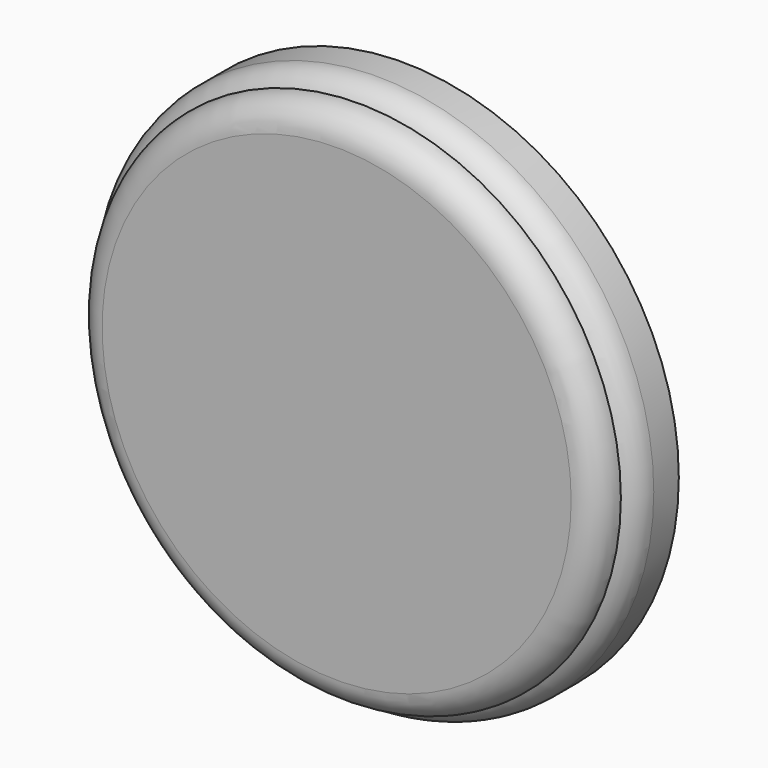
from build123d import *

# Parameters (mm, degrees)
F0_R     = 50
F1_DEPTH = 10
F2_R     = 47.5
F3_DEPTH = 5


# Not quite as in the source:
# - a fillet or chamfer that OpenCascade refuses, or shapes differently, is made with other operations: its cross-section is extruded or revolved along the edge and cut away or added


with BuildPart() as f1:
    # F0 (on Front) → F1 (new body)
    with BuildSketch(Plane.XZ):
        Circle(F0_R)
    extrude(amount=F1_DEPTH)

    # F2 (on face) → F3 (join)
    with BuildSketch(Plane.XZ.offset(10)):
        Circle(F2_R)
    extrude(amount=F3_DEPTH)

    # F4: fillet of radius 5 on 2 edges, made by hand

    # F4_s1 → F4_t2 (revolve, cut)
    with BuildSketch(Plane.XY):
        with BuildLine():
            ThreePointArc((50, -5.6698729811), (49.3301270189, -8.1698729811), (47.5, -10))
            Line((47.5, -10), (50, -10))
            Line((50, -10), (50, -5.6698729811))
        make_face()
    revolve(axis=Axis((0, -10, 0), (0, -1, 0)), mode=Mode.SUBTRACT)

    # F4_s3 → F4_t4 (revolve, cut)
    with BuildSketch(Plane.XY):
        with BuildLine():
            ThreePointArc((47.5, -10), (46.0355339059, -13.5355339059), (42.5, -15))
            Line((42.5, -15), (47.5, -15))
            Line((47.5, -15), (47.5, -10))
        make_face()
    revolve(axis=Axis((0, -15, 0), (0, -1, 0)), mode=Mode.SUBTRACT)


solid = f1.part
